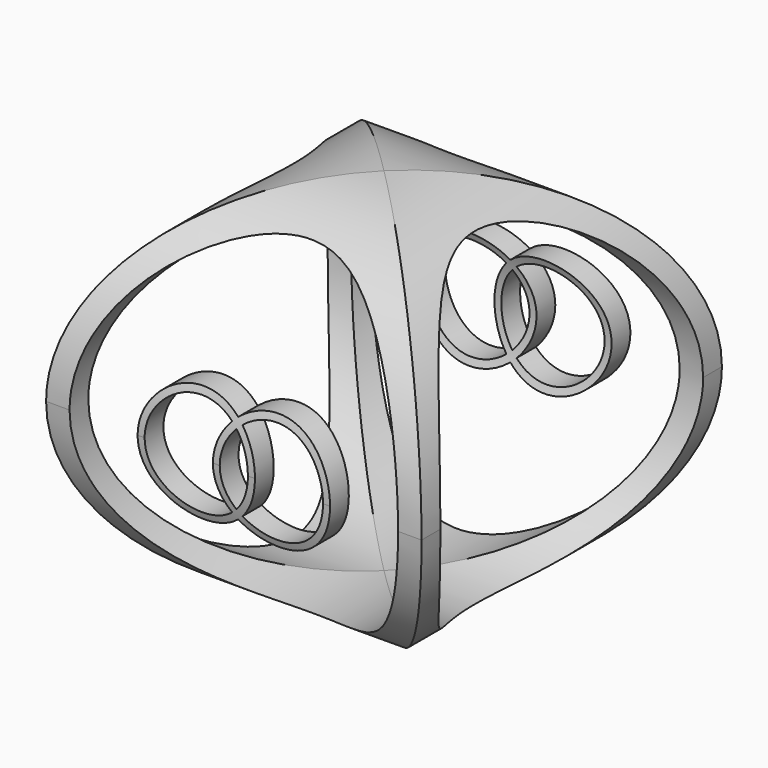
from build123d import *
from build123d import SkipClean  # not in build123d's __all__

# Parameters (mm, degrees)
F0_W       = 80
F0_H       = 80
F1_DEPTH   = 40
F1_FACE1_W = 80
F1_FACE1_H = 80
F3_DEPTH   = 90
F4_W       = 113.8921592288
F4_H       = 105.8337588391
F4_R       = 40
F5_DEPTH   = 50
F6_R       = 35
F7_DEPTH   = 75
F8_R       = 35
F9_DEPTH   = 75
F11_DEPTH  = 75


with BuildPart() as f1:
    # F0 (on Top) → F1 (new body, symmetric)
    with BuildSketch(Plane.XY):
        Rectangle(F0_W, F0_H)
    extrude(amount=F1_DEPTH, both=True)

    # F2 (on face) + F1_face1 (on face) → F3 (cut)
    with BuildSketch(Plane.YZ.offset(40)):
        with BuildLine():
            ThreePointArc((-40, 0), (-28.2842712475, 28.2842712475), (0, 40))
            Line((0, 40), (-40, 40))
            Line((-40, 40), (-40, 0))
        make_face()
        with BuildLine():
            ThreePointArc((0, 40), (28.2842712475, 28.2842712475), (40, 0))
            Line((40, 0), (40, 40))
            Line((40, 40), (0, 40))
        make_face()
        with BuildLine():
            Line((40, -40), (40, 0))
            ThreePointArc((40, 0), (28.2842712475, -28.2842712475), (0, -40))
            Line((0, -40), (40, -40))
        make_face()
        with BuildLine():
            Line((-40, -40), (0, -40))
            ThreePointArc((0, -40), (-28.2842712475, -28.2842712475), (-40, 0))
            Line((-40, 0), (-40, -40))
        make_face()
    with BuildSketch(Plane(origin=(-40, 0, 0), x_dir=(0, -1, 0), z_dir=(-1, 0, 0))):
        Rectangle(F1_FACE1_W, F1_FACE1_H)
    extrude(amount=-F3_DEPTH, dir=(1, 0, 0), mode=Mode.SUBTRACT)

    # F4 (on Front) → F5 (cut, symmetric)
    with BuildSketch(Plane.XZ):
        with Locations((3.1338229844, 0.2686137127)):
            Rectangle(F4_W, F4_H)
        Circle(F4_R, mode=Mode.SUBTRACT)
    extrude(amount=F5_DEPTH, both=True, mode=Mode.SUBTRACT)

    # F6 (on Front) → F7 (cut, symmetric)
    with BuildSketch(Plane.XZ):
        Circle(F6_R)
        with BuildLine():
            ThreePointArc((0, -9.6046863561), (-20.5, 0), (0, 9.6046863561))
            ThreePointArc((0, 9.6046863561), (13.3033008589, 11.3192314227), (20.5, 0))
            ThreePointArc((20.5, 0), (13.3033008589, -11.3192314227), (0, -9.6046863561))
        make_face(mode=Mode.SUBTRACT)
    extrude(amount=F7_DEPTH, both=True, mode=Mode.SUBTRACT)

    # F8 (on Right) → F9 (cut, symmetric)
    with BuildSketch(Plane.YZ):
        Circle(F8_R)
    extrude(amount=F9_DEPTH, both=True, mode=Mode.SUBTRACT)

    # F10 (on Front) → F11 (cut, symmetric)
    with BuildSketch(Plane.XZ):
        with BuildLine():
            ThreePointArc((0, 7.5498344353), (-3, 0), (0, -7.5498344353))
            ThreePointArc((0, -7.5498344353), (3, 0), (0, 7.5498344353))
        make_face()
        with BuildLine():
            ThreePointArc((1.1015625, 8.5680546251), (4.5, 0), (1.1015625, -8.5680546251))
            ThreePointArc((1.1015625, -8.5680546251), (19, 0), (1.1015625, 8.5680546251))
        make_face()
        with BuildLine():
            ThreePointArc((-1.0714844426, -8.5437504745), (-4.4614406135, 0), (-1.0714844426, 8.5437504745))
            ThreePointArc((-1.0714844426, 8.5437504745), (-19, 0), (-1.0714844426, -8.5437504745))
        make_face()
    with SkipClean():  # cleaning this boolean's faces spoils the solid; the shape is the same uncleaned
        extrude(amount=F11_DEPTH, both=True, mode=Mode.SUBTRACT)


solid = f1.part
